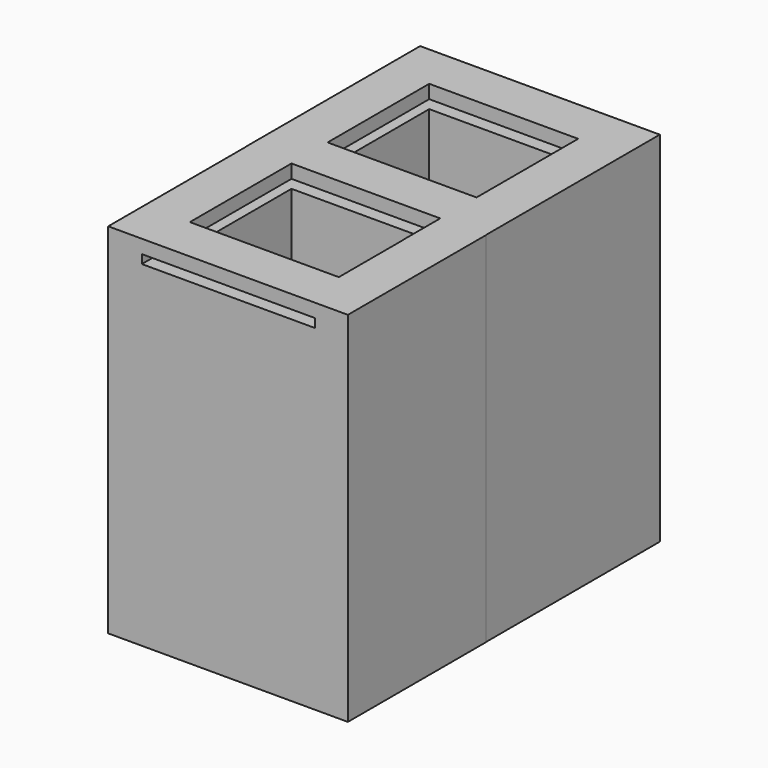
from build123d import *

# Parameters (mm, degrees)
F1_DEPTH      = 125.4125
F2_T          = -15.875
F4_DEPTH      = 125.4125
F5_T          = -15.875
F7_W          = 60.6690326877
F7_H          = 3.0675412395
F8_DEPTH      = 182.626
F8_DEPTH_BACK = 25.4


# Not quite as in the source:
# - a shell that OpenCascade refuses in one call is made with other operations: the cavity is built on its own and cut out


with BuildPart() as f1:
    # F0 (on Top) → F1 (new body)
    with BuildSketch(Plane.XY):
        Polygon((41.9354, 38.1), (-41.9354, 38.1), (-41.9354, -38.1), align=None)
        Polygon((41.9354, -38.1), (41.9354, 38.1), (-41.9354, -38.1), align=None)
    extrude(amount=F1_DEPTH)

    # F2
    f2_openings = [f1.faces().sort_by_distance(p)[0] for p in [
        (0, 0, 125.4125),
    ]]
    offset(amount=F2_T, openings=f2_openings)

    # F3 (on Top) → F4 (join)
    with BuildSketch(Plane.XY):
        Polygon((42.0021460263, -98.425), (-41.8686539737, -38.1), (-41.8686539737, -98.425), align=None)
        Polygon((42.0021460263, -38.1), (-41.8686539737, -38.1), (42.0021460263, -98.425), align=None)
    extrude(amount=F4_DEPTH)

    # F5: a shell. OpenCascade refuses it in one call, so the cavity is built on its own and cut out:
    # the body offset inwards by the wall thickness, plus a prism from it out through each open face.
    f5_core = offset(f1.part, amount=F5_T, kind=Kind.INTERSECTION, mode=Mode.PRIVATE)
    f5_exits = [f5_core.faces().sort_by_distance(p)[0] for p in [
        (0.054837, -60.331537, 109.5375),
    ]]
    add(f5_core, mode=Mode.SUBTRACT)
    extrude(f5_exits, amount=-F5_T, mode=Mode.SUBTRACT)

    # F7 (on offset) → F8 (cut, two sides)
    with BuildSketch(Plane.XZ.offset(123.825)) as f8_sk:
        with Locations((0.2376296824, 119.1418357193)):
            Rectangle(F7_W, F7_H)
    extrude(amount=-F8_DEPTH, mode=Mode.SUBTRACT)
    extrude(f8_sk.sketch, amount=F8_DEPTH_BACK, mode=Mode.SUBTRACT)


solid = f1.part
